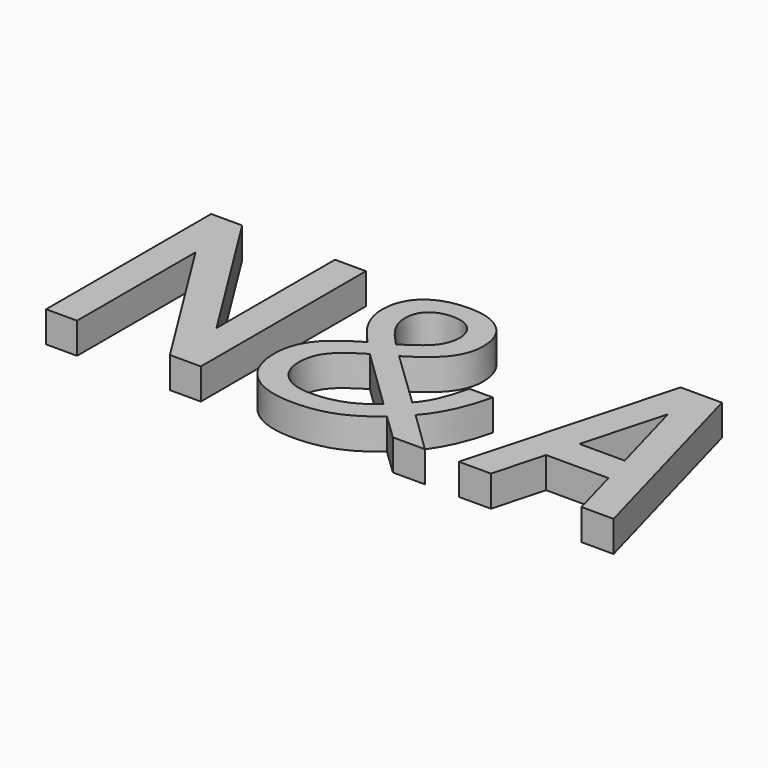
from build123d import *

# Parameters (mm, degrees)
F1_DEPTH     = 60
F0_TEXT_SIZE = 555.5555555556
F2_DEPTH     = 60


# Not quite as in the source:
# - Text() gives the source's letters only with a copy of the font that has no kerning and outlines rounded to 1/6400 em; it was checked with that copy


with BuildPart() as f1:
    # F0 (on Top) → F1 (new body)
    with BuildSketch(Plane.XY):
        Polygon((240, 112.941707368), (240, 0), (300, 0), (300, 400), (240, 400), align=None)
        Polygon((60, 400), (60, 287.058292632), (240, 0), (240, 112.941707368), align=None)
        Polygon((0, 400), (0, 0), (60, 0), (60, 287.058292632), (60, 400), align=None)
    extrude(amount=F1_DEPTH)

    # F0 (on Top) → F2 (join)
    with BuildSketch(Plane.XY):
        Polygon((0, 400), (0, 0), (60, 0), (60, 287.058292632), (60, 400), align=None)
        Polygon((60, 400), (60, 287.058292632), (240, 0), (240, 112.941707368), align=None)
        Polygon((240, 112.941707368), (240, 0), (300, 0), (300, 400), (240, 400), align=None)
        Polygon((990, 400), (910, 400), (800, 0), (862.2274055381, 0), (889.613702769, 99.5865353853), (906.113702769, 159.5865353853), (950, 319.1730707706), (993.886297231, 159.5865353853), (1010.386297231, 99.5865353853), (1037.7725944619, 0), (1100, 0), align=None)
        Polygon((906.113702769, 159.5865353853), (889.613702769, 99.5865353853), (1010.386297231, 99.5865353853), (993.886297231, 159.5865353853), align=None)
        with Locations((329.7743055556, 0)):
            Text('&', F0_TEXT_SIZE, font='Open Sans', text_align=(TextAlign.LEFT, TextAlign.BOTTOM))
    extrude(amount=F2_DEPTH)


solid = f1.part
